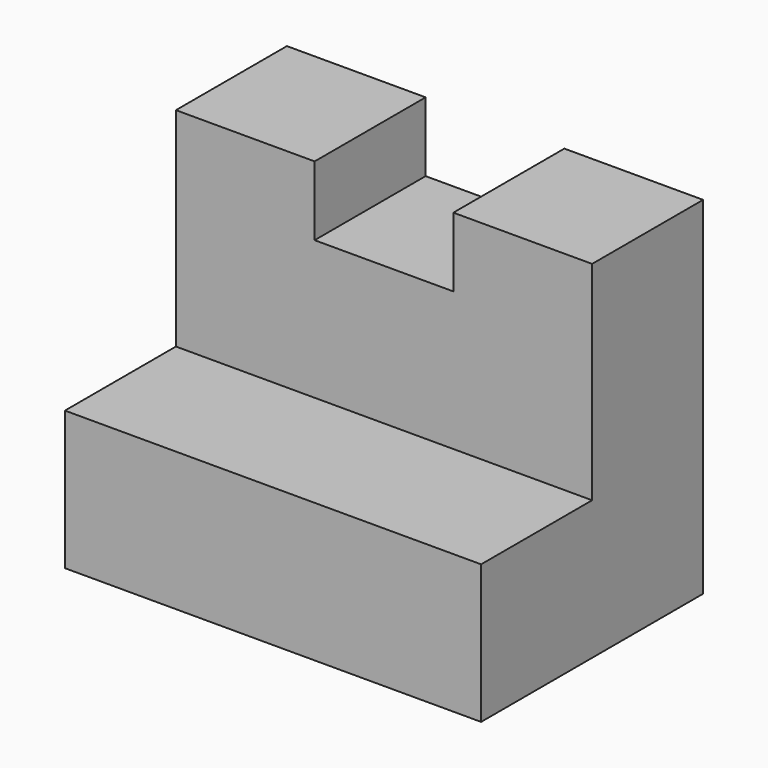
from build123d import *

# Parameters (mm, degrees)
F1_DEPTH = 38.1
F2_W     = 12.7
F2_H     = 6.35
F3_DEPTH = 12.7


# Not quite as in the source:
# - a feature names something its author has since deleted; it is built from what else it names


with BuildPart() as f1:
    # F0 (on Right) → F1 (new body)
    with BuildSketch(Plane.YZ):
        Polygon((-23.0481477177, 0), (-23.0481477177, 31.75), (-35.7481477177, 31.75), (-35.7481477177, 12.7), (-48.4481477177, 12.7), (-48.4481477177, 0), align=None)
    extrude(amount=F1_DEPTH)

    # F2 (on face) → F3 (cut)
    with BuildSketch(Plane.XZ.offset(35.7481477177)):
        with Locations((19.05, 28.575)):
            Rectangle(F2_W, F2_H)
    extrude(amount=-F3_DEPTH, mode=Mode.SUBTRACT)


solid = f1.part
